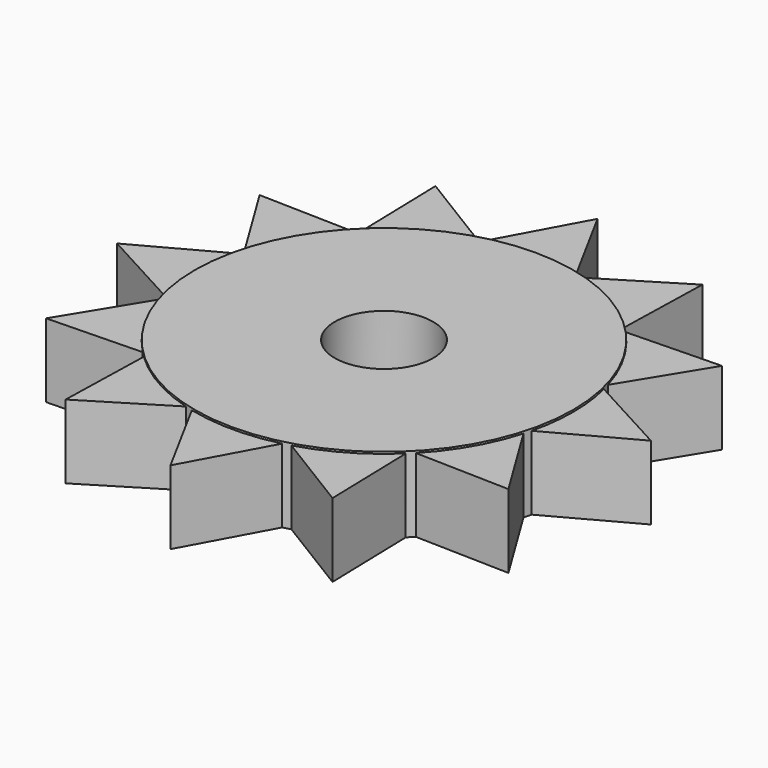
from build123d import *

# Parameters (mm, degrees)
F0_R            = 50
F1_DEPTH        = 20
F2_R            = 13
F3_DEPTH        = 20
F5_DEPTH        = 19.5
F5_COPIES_COUNT = 12


# Not quite as in the source:
# - a pattern or mirror of a feature is missing from the dataset's text; its kind, count and spacing are read off the source's solid


with BuildPart() as f1:
    # F0 (on Top) → F1 (new body)
    with BuildSketch(Plane.XY):
        Circle(F0_R)
    extrude(amount=F1_DEPTH)

    # F2 (on Top) → F3 (cut)
    with BuildSketch(Plane.XY):
        Circle(F2_R)
    extrude(amount=F3_DEPTH, mode=Mode.SUBTRACT)

    # F4 (on Top) → F5 (join)
    with BuildSketch(Plane.XY):
        with BuildLine():
            Line((0, 70.5249483342), (-11.9310349513, 48.55564236))
            ThreePointArc((-11.9310349513, 48.55564236), (0, 50), (11.9310349513, 48.55564236))
            Line((11.9310349513, 48.55564236), (0, 70.5249483342))
        make_face()
    f5 = extrude(amount=F5_DEPTH)

    # F5_copies: F5 ×12 about axis
    f5_copies_axis = Axis((0, 0, 0), (0, 0, 1))
    for i in range(1, F5_COPIES_COUNT):
        add(f5.rotate(f5_copies_axis, i * 360 / F5_COPIES_COUNT))


solid = f1.part
